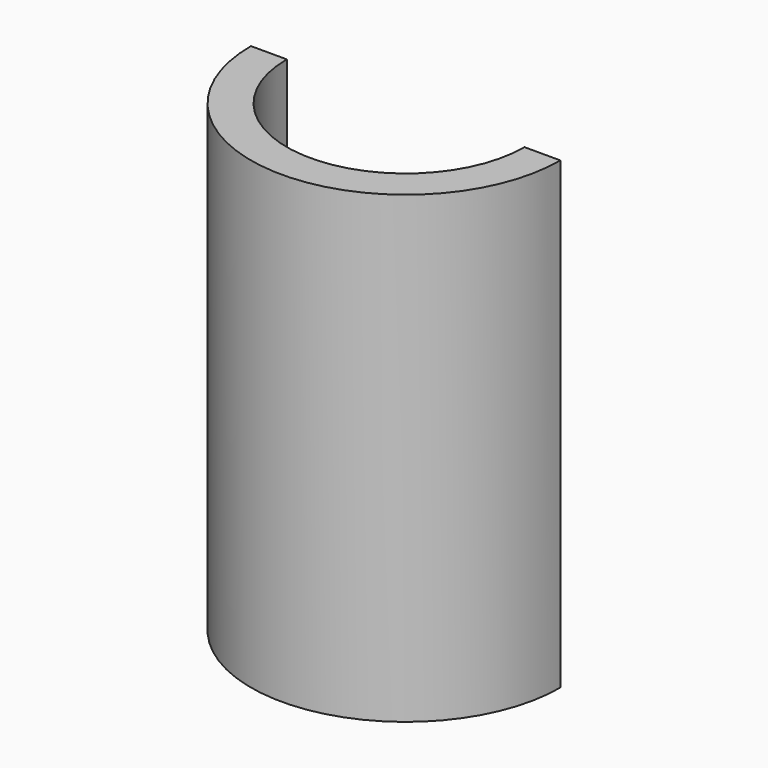
from build123d import *

# Parameters (mm, degrees)
F1_DEPTH = 228.6


with BuildPart() as f1:
    # F0 (on Top) → F1 (new body)
    with BuildSketch(Plane.XY):
        with BuildLine():
            ThreePointArc((-76.212198746, 0), (0, -76.212198746), (76.212198746, 0))
            Line((76.212198746, 0), (58.5254982315, 0))
            ThreePointArc((58.5254982315, 0), (0, -58.5254982315), (-58.5254982315, 0))
            Line((-58.5254982315, 0), (-76.212198746, 0))
        make_face()
    extrude(amount=F1_DEPTH)


solid = f1.part
